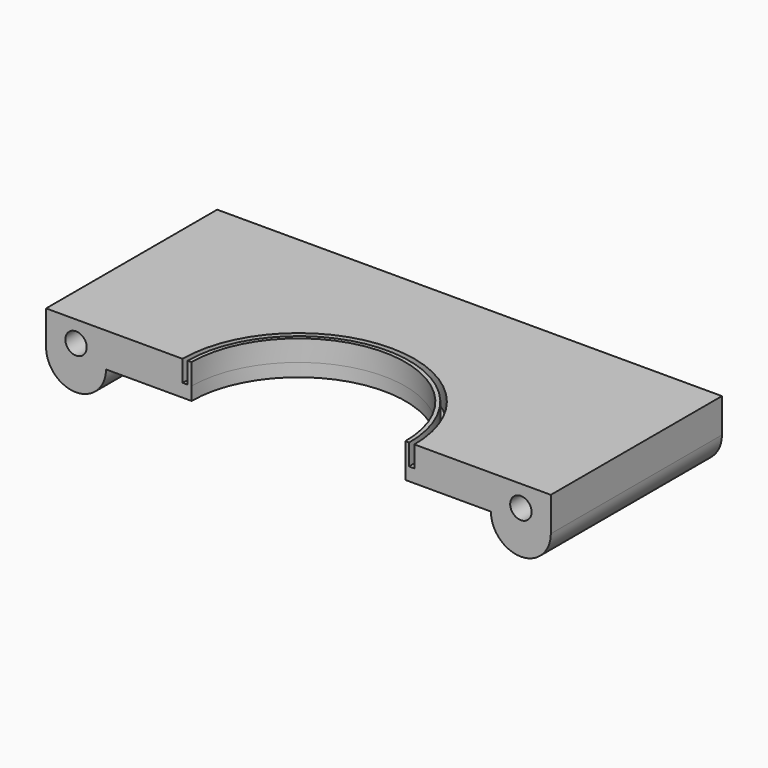
from build123d import *

# Parameters (mm, degrees)
F0_R     = 2.5
F1_DEPTH = 50
F2_R     = 25
F3_DEPTH = 25
F4_DEPTH = 50
F5_DEPTH = 25
F6_R     = 27.1
F6_R_2   = 25.9
F7_DEPTH = 5
F8_DEPTH = 25


# Not quite as in the source:
# - a feature names something its author has since deleted; it is built from what else it names


with BuildPart() as f1:
    # F0 (on Front) → F1 (new body)
    with BuildSketch(Plane.XZ):
        Polygon((90, 4.9383143896), (0, 4.9383143896), (0, -0.0616856104), (0, -3.0616856104), (90, -3.0616856104), (90, -0.0616856104), align=None)
        with BuildLine():
            Line((0, -0.0616856104), (0, 4.9383143896))
            Line((0, 4.9383143896), (-14, 4.9383143896))
            Line((-14, 4.9383143896), (-14, -3.0616856104))
            ThreePointArc((-14, -3.0616856104), (-7, -10.0616856104), (0, -3.0616856104))
            Line((0, -3.0616856104), (0, -0.0616856104))
        make_face()
        with Locations((-7, 0)):
            Circle(F0_R, mode=Mode.SUBTRACT)
    extrude(amount=F1_DEPTH)

    # F2 (on Top) → F3 (cut)
    with BuildSketch(Plane.XY):
        with Locations((45, -50)):
            Circle(F2_R)
    extrude(amount=-F3_DEPTH, mode=Mode.SUBTRACT)

    # F0 (on Front) → F4 (join)
    with BuildSketch(Plane.XZ):
        Polygon((90, 4.9383143896), (0, 4.9383143896), (0, -0.0616856104), (0, -3.0616856104), (90, -3.0616856104), (90, -0.0616856104), align=None)
        with BuildLine():
            Line((0, -0.0616856104), (0, 4.9383143896))
            Line((0, 4.9383143896), (-14, 4.9383143896))
            Line((-14, 4.9383143896), (-14, -3.0616856104))
            ThreePointArc((-14, -3.0616856104), (-7, -10.0616856104), (0, -3.0616856104))
            Line((0, -3.0616856104), (0, -0.0616856104))
        make_face()
        with Locations((-7, 0)):
            Circle(F0_R, mode=Mode.SUBTRACT)
        with BuildLine():
            Line((104, 4.9383143896), (90, 4.9383143896))
            Line((90, 4.9383143896), (90, -0.0616856104))
            Line((90, -0.0616856104), (90, -3.0616856104))
            ThreePointArc((90, -3.0616856104), (97, -10.0616856104), (104, -3.0616856104))
            Line((104, -3.0616856104), (104, -0.0616856104))
            Line((104, -0.0616856104), (104, 4.9383143896))
        make_face()
        with Locations((97, -0.0616856104)):
            Circle(F0_R, mode=Mode.SUBTRACT)
    extrude(amount=F4_DEPTH)

    # F2 (on Top) → F5 (cut)
    with BuildSketch(Plane.XY):
        with Locations((45, -50)):
            Circle(F2_R)
    extrude(amount=-F5_DEPTH, mode=Mode.SUBTRACT)

    # F6 (on Top) → F7 (cut)
    with BuildSketch(Plane.XY):
        with Locations((45, -50)):
            Circle(F6_R)
        with Locations((45, -50)):
            Circle(F6_R_2, mode=Mode.SUBTRACT)
    extrude(amount=F7_DEPTH, mode=Mode.SUBTRACT)

    # F2 (on Top) → F8 (cut)
    with BuildSketch(Plane.XY):
        with Locations((45, -50)):
            Circle(F2_R)
    extrude(amount=F8_DEPTH, mode=Mode.SUBTRACT)


solid = f1.part
